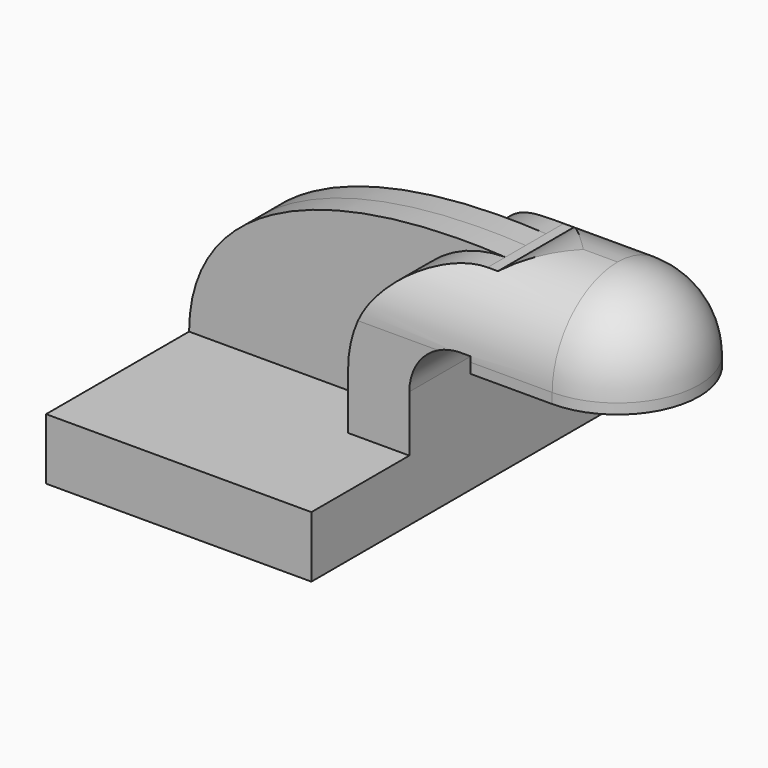
from build123d import *

# Parameters (mm, degrees)
F1_DEPTH    = 63.5
F0_W        = 25.4
F0_H        = 19.05
F0_H_2      = 4.7498
F0_H_3      = 4.7752
F2_DEPTH    = 25.4
F3_DEPTH    = 7.8867
F5_T1_DEPTH = 124.7474881183
F5_T3_DEPTH = 88.9
F5_T6_ANGLE = 180


# Not quite as in the source:
# - a fillet or chamfer that OpenCascade refuses, or shapes differently, is made with other operations: its cross-section is extruded or revolved along the edge and cut away or added


with BuildPart() as f1:
    # F0 (on Front) → F1 (new body, symmetric)
    with BuildSketch(Plane.XZ):
        Polygon((22.225, 9.525), (-41.275, 9.525), (-41.275, -9.525), (41.275, -9.525), (41.275, 9.525), align=None)
    extrude(amount=F1_DEPTH, both=True)

    # F0 (on Front) → F2 (join, symmetric)
    with BuildSketch(Plane.XZ):
        with BuildLine():
            Line((22.225, 27.0002), (22.225, 9.525))
            Line((22.225, 9.525), (41.275, 9.525))
            Line((41.275, 9.525), (41.275, 27.0002))
            ThreePointArc((41.275, 27.0002), (45.9246798487, 38.2255201513), (57.15, 42.8752))
            Line((57.15, 42.8752), (60.325, 42.8752))
            Line((60.325, 42.8752), (60.325, 61.9252))
            Line((60.325, 61.9252), (57.15, 61.9252))
            ThreePointArc((57.15, 61.9252), (32.4542956671, 51.6959043329), (22.225, 27.0002))
        make_face()
        with Locations((73.025, 52.4002)):
            Rectangle(F0_W, F0_H)
        with Locations((73.025, 64.3001)):
            Rectangle(F0_W, F0_H_2)
        with Locations((73.025, 40.4876)):
            Rectangle(F0_W, F0_H_3)
    extrude(amount=F2_DEPTH, both=True)

    # F0 (on Front) → F3 (join, symmetric)
    with BuildSketch(Plane.XZ):
        with BuildLine():
            add(Edge.make_bspline(
                [(-41.275, 9.525), (-41.0557202995, 48.5295318067), (2.8826263733, 65.0303959846), (57.15, 61.9252)],
                knots=[0, 0, 0, 0, 111.5045361635, 111.5045361635, 111.5045361635, 111.5045361635], degree=3))
            Line((-41.275, 9.525), (22.225, 9.525))
            Line((22.225, 9.525), (22.225, 27.0002))
            ThreePointArc((22.225, 27.0002), (32.4542956671, 51.6959043329), (57.15, 61.9252))
        make_face()
    extrude(amount=F3_DEPTH, both=True)

    # F0 (on Front) → F4 (revolve)
    with BuildSketch(Plane.XZ):
        Polygon((85.725, 66.675), (85.725, 61.9252), (85.725, 42.8752), (85.725, 38.1), (111.125, 38.1), (111.125, 66.675), align=None)
    revolve(axis=Axis((85.725, 0, 52.3875), (0, 0, 1)))

    # F5: fillet of radius 25.4 on 4 edges, made by hand

    # F5_s2 → F5_t1 (cut)
    with BuildSketch(Plane.XZ.offset(-62.3737440591)):
        with BuildLine():
            ThreePointArc((60.325, 61.9252), (67.3477441191, 65.4584145645), (75.1144976237, 66.675))
            Line((75.1144976237, 66.675), (60.325, 66.675))
            Line((60.325, 66.675), (60.325, 61.9252))
        make_face()
    extrude(amount=F5_T1_DEPTH, mode=Mode.SUBTRACT)

    # F5_s4 → F5_t3 (cut)
    with BuildSketch(Plane.YZ.offset(-3.175)):
        with BuildLine():
            ThreePointArc((-25.4, 41.275), (-17.9605122421, 59.2355122421), (0, 66.675))
            Line((0, 66.675), (-25.4, 66.675))
            Line((-25.4, 66.675), (-25.4, 41.275))
        make_face()
        with BuildLine():
            ThreePointArc((0, 66.675), (17.9605122421, 59.2355122421), (25.4, 41.275))
            Line((25.4, 41.275), (25.4, 66.675))
            Line((25.4, 66.675), (0, 66.675))
        make_face()
    extrude(amount=F5_T3_DEPTH, mode=Mode.SUBTRACT)

    # F5_s5 → F5_t6 (revolve, cut)
    with BuildSketch(Plane.YZ.offset(85.725)):
        with BuildLine():
            ThreePointArc((0, 66.675), (17.9605122421, 59.2355122421), (25.4, 41.275))
            Line((25.4, 41.275), (25.4, 66.675))
            Line((25.4, 66.675), (0, 66.675))
        make_face()
    revolve(axis=Axis((85.725, 0, 66.675), (0, 0, -1)), revolution_arc=F5_T6_ANGLE, mode=Mode.SUBTRACT)


solid = f1.part
